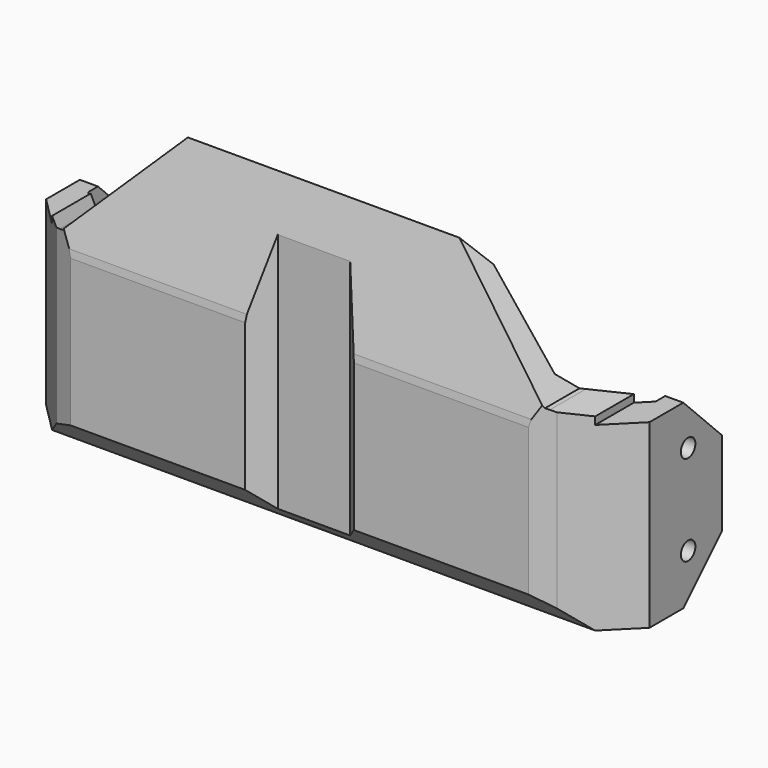
from build123d import *

# Parameters (mm, degrees)
F1_DEPTH      = 30
F2_SIZE       = 10
F4_DEPTH      = 50
F5_DEPTH      = 20
F6_DEPTH      = 25
F8_DEPTH      = 25.001
F9_DEPTH      = 25
F11_W         = 8
F11_H         = 3
F12_DEPTH     = 50.001
F13_T1_DEPTH  = 61.7168298797
F13_T3_DEPTH  = 40.0719817161
F13_T5_DEPTH  = 45.2357066129
F13_T10_DEPTH = 64.7177203375
F13_T15_DEPTH = 64.7177203375
F14_T1_DEPTH  = 56.7168298797
F14_T3_DEPTH  = 45.2357066129
F14_T5_DEPTH  = 35.0719817161
F15_R         = 1.5
F16_DEPTH     = 100.001
F18_SIZE      = 8
F19_SIZE      = 2.99999


# Not quite as in the source:
# - a fillet or chamfer that OpenCascade refuses, or shapes differently, is made with other operations: its cross-section is extruded or revolved along the edge and cut away or added
# - a fillet or chamfer is up to 0.001 mm smaller than in the source, because OpenCascade refuses the exact size


with BuildPart() as f1:
    # F0 (on Top) → F1 (new body)
    with BuildSketch(Plane.XY):
        Polygon((-47, 20), (-50, 20), (-50, -5), (50, -5), (50, 20), (47, 20), (47, 0), (-47, 0), align=None)
    extrude(amount=F1_DEPTH)

    # F2
    f2_edges = [f1.edges().sort_by_distance(p)[0] for p in [
        (-47, 0, 15),
        (47, 0, 15),
        (-50, -5, 15),
        (50, -5, 15),
    ]]
    chamfer(f2_edges, length=F2_SIZE)

    # F3 (on Right) → F4 (join, symmetric)
    with BuildSketch(Plane.YZ):
        Polygon((-5, 30), (0, 30), (2.9104275004, 49.2723931249), (0, 50), align=None)
    extrude(amount=F4_DEPTH, both=True)

    # F5 (add): faces of the model
    f5_faces = [f1.faces().sort_by_distance(p)[0] for p in [
        (46.0427350427, 7.6495726496, 30),
        (-46.0427350427, 7.6495726496, 30),
    ]]
    extrude(f5_faces, amount=F5_DEPTH)

    # F6 (cut): faces of the model
    f6_faces = [f1.faces().sort_by_distance(p)[0] for p in [
        (46.1111111111, -2.7777777778, 30),
        (-46.1111111111, -2.7777777778, 30),
    ]]
    extrude(f6_faces, amount=-F6_DEPTH, mode=Mode.SUBTRACT)

    # F7 (on face) → F8 (cut, through all)
    with BuildSketch(Plane.XZ.offset(5)):
        Polygon((40.5882352941, 32.3529411765), (45, 50), (37, 50), (22.5, 50), (40, 32.5), align=None)
        Polygon((45, 31.25), (45, 50), (40.5882352941, 32.3529411765), align=None)
        Polygon((45, 50), (47.9104275004, 49.2723931249), (45.1819017188, 31.2045245703), (50, 30), (50, 50), align=None)
    extrude(amount=-F8_DEPTH, mode=Mode.SUBTRACT)

    # F9 (cut): a face of the model
    f9_faces = [f1.faces().sort_by_distance(p)[0] for p in [
        (46.0411372728, 0, 41.900989059),
    ]]
    extrude(f9_faces, amount=-F9_DEPTH, mode=Mode.SUBTRACT)

    # F10: F1 across plane


with BuildPart() as f1_1:
    add(f1.part)
    add(f1.part.mirror(Plane.YZ), mode=Mode.INTERSECT)

    # F11 (on face) → F12 (cut, through all)
    with BuildSketch(Plane(origin=(0, 0, 0), x_dir=(1, 0, 0), z_dir=(0, 0, -1))):
        with Locations((0, 3.5)):
            Rectangle(F11_W, F11_H)
    extrude(amount=-F12_DEPTH, mode=Mode.SUBTRACT)

    # F13: chamfer of 5 on 5 edges, made by hand

    # F13_s2 → F13_t1 (cut)
    with BuildSketch(Plane.YZ.offset(-52.8584149398)):
        Polygon((0, 0), (-5, 5), (-5, 0), align=None)
    extrude(amount=F13_T1_DEPTH, mode=Mode.SUBTRACT)

    # F13_s4 → F13_t3 (cut)
    with BuildSketch(Plane.YZ.offset(-42.0359908581)):
        Polygon((-5, 29.3844718719), (-4.8507125007, 30.5971499971), (-5, 30), align=None)
    extrude(amount=F13_T3_DEPTH, mode=Mode.SUBTRACT)

    # F13_s6 → F13_t5 (cut)
    with BuildSketch(Plane.XY.offset(-5.6428543011)):
        Polygon((-41.4644660941, -3.5355339059), (-37.9289321881, -5), (-40, -5), align=None)
    extrude(amount=F13_T5_DEPTH, mode=Mode.SUBTRACT)


with BuildPart() as f13_tool8:
    # F13_s9 → F13_t10 (new body)
    with BuildSketch(Plane.XY.offset(-12.8584149398)):
        Polygon((9, -5), (4, 0), (4, -5), align=None)
    extrude(amount=F13_T10_DEPTH)

    split(bisect_by=Plane.XZ.offset(2), keep=Keep.TOP)


with BuildPart() as f1_2:
    add(f1_1.part)

    # F13_t7: cut F13_tool8
    add(f13_tool8.part, mode=Mode.SUBTRACT)


with BuildPart() as f13_tool13:
    # F13_s14 → F13_t15 (new body)
    with BuildSketch(Plane.XY.offset(-12.8584149398)):
        Polygon((-4, 0), (-9, -5), (-4, -5), align=None)
    extrude(amount=F13_T15_DEPTH)

    split(bisect_by=Plane.XZ.offset(2), keep=Keep.TOP)


with BuildPart() as f1_3:
    add(f1_2.part)

    # F13_t12: cut F13_tool13
    add(f13_tool13.part, mode=Mode.SUBTRACT)

    # F14: chamfer of 5 on 3 edges, made by hand

    # F14_s2 → F14_t1 (cut)
    with BuildSketch(Plane.YZ.offset(-3.8584149398)):
        Polygon((-5, 5), (0, 0), (-5, 0), align=None)
    extrude(amount=F14_T1_DEPTH, mode=Mode.SUBTRACT)

    # F14_s4 → F14_t3 (cut)
    with BuildSketch(Plane.XY.offset(-5.6428543011)):
        Polygon((41.4644660941, -3.5355339059), (37.9289321881, -5), (40, -5), align=None)
    extrude(amount=F14_T3_DEPTH, mode=Mode.SUBTRACT)

    # F14_s6 → F14_t5 (cut)
    with BuildSketch(Plane.YZ.offset(6.9640091419)):
        Polygon((-5, 29.3844718719), (-4.8507125007, 30.5971499971), (-5, 30), align=None)
    extrude(amount=F14_T5_DEPTH, mode=Mode.SUBTRACT)

    # F15 (on face) → F16 (cut, through all)
    with BuildSketch(Plane(origin=(-50, 0, 0), x_dir=(0, -1, 0), z_dir=(-1, 0, 0))):
        with Locations((-13, 23)):
            Circle(F15_R)
        with Locations((-13, 8)):
            Circle(F15_R)
    extrude(amount=-F16_DEPTH, mode=Mode.SUBTRACT)

    # F17: F1 across plane


with BuildPart() as f1_4:
    add(f1_3.part)
    add(f1_3.part.mirror(Plane.YZ), mode=Mode.INTERSECT)

    # F18
    f18_edges = [f1_4.edges().sort_by_distance(p)[0] for p in [
        (48.5, 20, 0),
        (-48.5, 20, 0),
        (-48.5, 20, 30),
        (48.5, 20, 30),
    ]]
    chamfer(f18_edges, length=F18_SIZE)

    # F19 (size 3 in the source; OpenCascade refuses exactly that, so slightly less here)
    f19_edges = [f1_4.edges().sort_by_distance(p)[0] for p in [
        (0, 2.910428, 49.272393),
    ]]
    chamfer(f19_edges, length=F19_SIZE)


solid = f1_4.part
